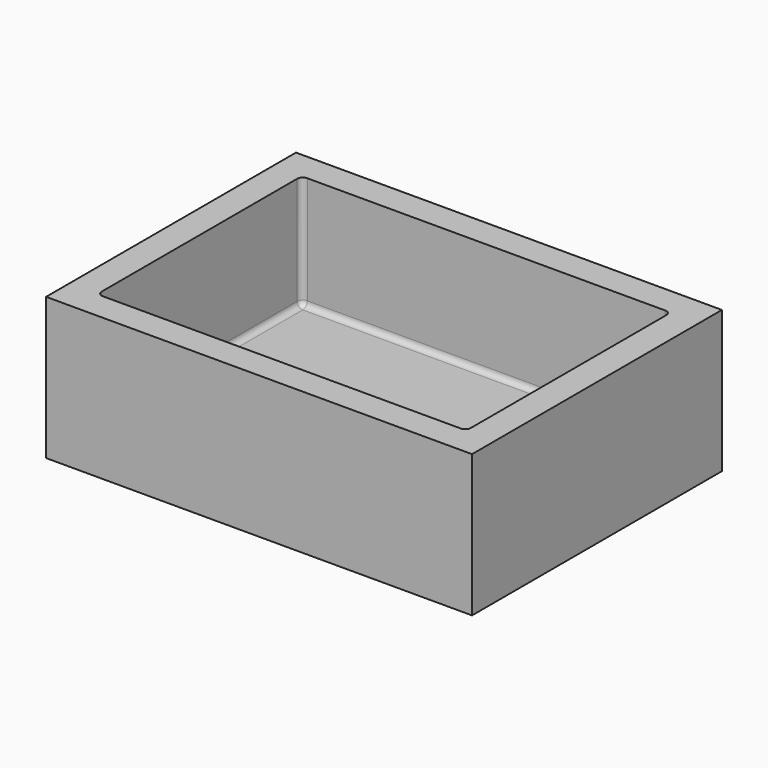
from build123d import *

# Parameters (mm, degrees)
F0_W         = 65
F0_H         = 45
F1_DEPTH     = 20
F2_T         = 5
F3_T1_DEPTH  = 19
F3_T3_DEPTH  = 63
F3_T5_DEPTH  = 43
F3_S9_W      = 1
F3_S9_H      = 1
F3_T10_DEPTH = 1
F3_S15_W     = 1
F3_S15_H     = 1
F3_T16_DEPTH = 1
F3_S21_W     = 1
F3_S21_H     = 1
F3_T22_DEPTH = 1
F3_S27_W     = 1
F3_S27_H     = 1
F3_T28_DEPTH = 1


# Not quite as in the source:
# - a fillet or chamfer that OpenCascade refuses, or shapes differently, is made with other operations: its cross-section is extruded or revolved along the edge and cut away or added


with BuildPart() as f1:
    # F0 (on Top) → F1 (new body)
    with BuildSketch(Plane.XY):
        Rectangle(F0_W, F0_H)
    extrude(amount=F1_DEPTH)

    # F2
    f2_openings = [f1.faces().sort_by_distance(p)[0] for p in [
        (0, 0, 20),
    ]]
    offset(amount=F2_T, openings=f2_openings, kind=Kind.INTERSECTION)

    # F3: fillet of radius 1 on 8 edges, made by hand

    # F3_s2 → F3_t1 (join)
    with BuildSketch(Plane.XY.offset(1)):
        with BuildLine():
            ThreePointArc((31.5, 22.5), (32.2071067812, 22.2071067812), (32.5, 21.5))
            Line((32.5, 21.5), (32.5, 22.5))
            Line((32.5, 22.5), (31.5, 22.5))
        make_face()
        with BuildLine():
            ThreePointArc((-31.5, 22.5), (-32.2071067812, 22.2071067812), (-32.5, 21.5))
            Line((-32.5, 21.5), (-32.5, 22.5))
            Line((-32.5, 22.5), (-31.5, 22.5))
        make_face()
        with BuildLine():
            ThreePointArc((-32.5, -21.5), (-32.2071067812, -22.2071067812), (-31.5, -22.5))
            Line((-31.5, -22.5), (-32.5, -22.5))
            Line((-32.5, -22.5), (-32.5, -21.5))
        make_face()
        with BuildLine():
            ThreePointArc((31.5, -22.5), (32.2071067812, -22.2071067812), (32.5, -21.5))
            Line((32.5, -21.5), (32.5, -22.5))
            Line((32.5, -22.5), (31.5, -22.5))
        make_face()
    extrude(amount=F3_T1_DEPTH)

    # F3_s4 → F3_t3 (join)
    with BuildSketch(Plane.YZ.offset(-31.5)):
        with BuildLine():
            ThreePointArc((22.5, 1), (22.2071067812, 0.2928932188), (21.5, 0))
            Line((21.5, 0), (22.5, 0))
            Line((22.5, 0), (22.5, 1))
        make_face()
        with BuildLine():
            ThreePointArc((-22.5, 1), (-22.2071067812, 0.2928932188), (-21.5, 0))
            Line((-21.5, 0), (-22.5, 0))
            Line((-22.5, 0), (-22.5, 1))
        make_face()
    extrude(amount=F3_T3_DEPTH)

    # F3_s6 → F3_t5 (join)
    with BuildSketch(Plane.XZ.offset(-21.5)):
        with BuildLine():
            ThreePointArc((-32.5, 1), (-32.2071067812, 0.2928932188), (-31.5, 0))
            Line((-31.5, 0), (-32.5, 0))
            Line((-32.5, 0), (-32.5, 1))
        make_face()
        with BuildLine():
            ThreePointArc((32.5, 1), (32.2071067812, 0.2928932188), (31.5, 0))
            Line((31.5, 0), (32.5, 0))
            Line((32.5, 0), (32.5, 1))
        make_face()
    extrude(amount=F3_T5_DEPTH)


with BuildPart() as f3_tool8:
    # F3_s9 → F3_t10 (new body)
    with BuildSketch(Plane.XZ.offset(-21.5)):
        with Locations((32, 0.5)):
            Rectangle(F3_S9_W, F3_S9_H)
    extrude(amount=-F3_T10_DEPTH)

    # F3_s11 → F3_t12 (revolve, cut)
    with BuildSketch(Plane(origin=(31.5, 21.5, 1), x_dir=(-0.7071067812, 0, 0.7071067812), z_dir=(-0.7071067812, 0, -0.7071067812))):
        with BuildLine():
            ThreePointArc((0, -1), (1, 0), (0, 1))
            Line((0, 1), (0, -1))
        make_face()
    revolve(axis=Axis((31.5, 21.5, 1), (0, 1, 0)), mode=Mode.SUBTRACT)


with BuildPart() as f1_1:
    add(f1.part)

    # F3_t7: union F3_tool8
    add(f3_tool8.part)


with BuildPart() as f3_tool14:
    # F3_s15 → F3_t16 (new body)
    with BuildSketch(Plane.XZ.offset(-21.5)):
        with Locations((-32, 0.5)):
            Rectangle(F3_S15_W, F3_S15_H)
    extrude(amount=-F3_T16_DEPTH)

    # F3_s17 → F3_t18 (revolve, cut)
    with BuildSketch(Plane(origin=(-31.5, 21.5, 1), x_dir=(0.7071067812, 0, 0.7071067812), z_dir=(-0.7071067812, 0, 0.7071067812))):
        with BuildLine():
            ThreePointArc((0, -1), (1, 0), (0, 1))
            Line((0, 1), (0, -1))
        make_face()
    revolve(axis=Axis((-31.5, 21.5, 1), (0, 1, 0)), mode=Mode.SUBTRACT)


with BuildPart() as f1_2:
    add(f1_1.part)

    # F3_t13: union F3_tool14
    add(f3_tool14.part)


with BuildPart() as f3_tool20:
    # F3_s21 → F3_t22 (new body)
    with BuildSketch(Plane.YZ.offset(-31.5)):
        with Locations((-22, 0.5)):
            Rectangle(F3_S21_W, F3_S21_H)
    extrude(amount=-F3_T22_DEPTH)

    # F3_s23 → F3_t24 (revolve, cut)
    with BuildSketch(Plane(origin=(-31.5, -21.5, 1), x_dir=(0, 0.7071067812, 0.7071067812), z_dir=(0, -0.7071067812, 0.7071067812))):
        with BuildLine():
            ThreePointArc((0, -1), (1, 0), (0, 1))
            Line((0, 1), (0, -1))
        make_face()
    revolve(axis=Axis((-31.5, -21.5, 1), (-1, 0, 0)), mode=Mode.SUBTRACT)


with BuildPart() as f1_3:
    add(f1_2.part)

    # F3_t19: union F3_tool20
    add(f3_tool20.part)


with BuildPart() as f3_tool26:
    # F3_s27 → F3_t28 (new body)
    with BuildSketch(Plane.XZ.offset(21.5)):
        with Locations((32, 0.5)):
            Rectangle(F3_S27_W, F3_S27_H)
    extrude(amount=F3_T28_DEPTH)

    # F3_s29 → F3_t30 (revolve, cut)
    with BuildSketch(Plane(origin=(31.5, -21.5, 1), x_dir=(-0.7071067812, 0, 0.7071067812), z_dir=(0.7071067812, 0, 0.7071067812))):
        with BuildLine():
            ThreePointArc((0, -1), (1, 0), (0, 1))
            Line((0, 1), (0, -1))
        make_face()
    revolve(axis=Axis((31.5, -21.5, 1), (0, -1, 0)), mode=Mode.SUBTRACT)


with BuildPart() as f1_4:
    add(f1_3.part)

    # F3_t25: union F3_tool26
    add(f3_tool26.part)


solid = f1_4.part
